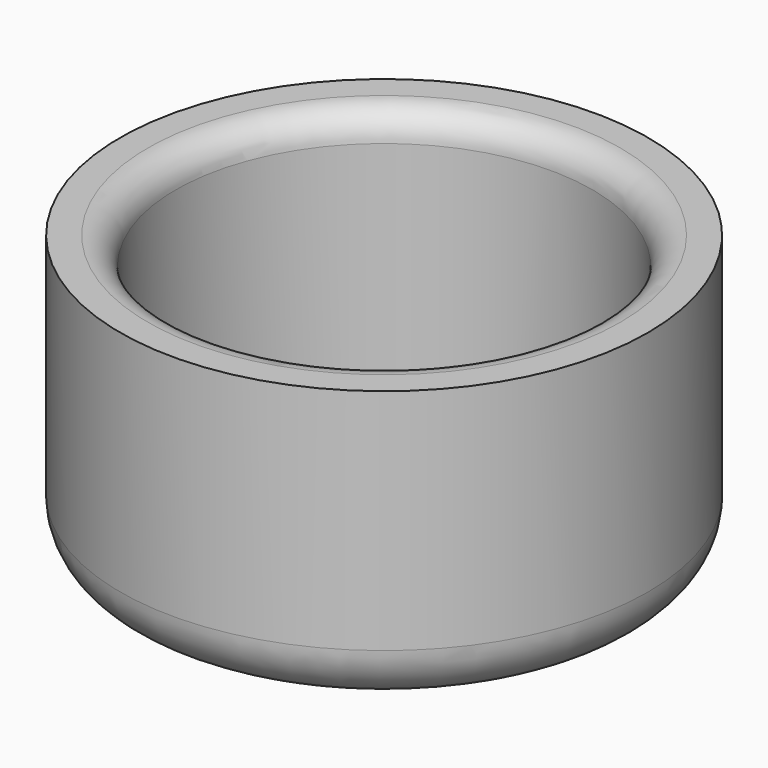
from build123d import *

# Parameters (mm, degrees)
F2_R         = 2
F3_R         = 1
F4_TEXT_SIZE = 3.9131940058
F5_DEPTH     = 1


# Not quite as in the source:
# - Text() gives the source's letters only with a copy of the font that has no kerning and outlines rounded to 1/6400 em; it was checked with that copy


with BuildPart() as f1:
    # F0 (on Front) → F1 (revolve)
    with BuildSketch(Plane.XZ):
        Polygon((7.5, 0), (0, 0), (0, -2), (9.5, -2), (9.5, 8.2183094201), (7.5, 8.2183094201), align=None)
    revolve(axis=Axis((0, 0, -1.6662292182), (0, 0, -1)))

    # F2
    f2_edges = [f1.edges().sort_by_distance(p)[0] for p in [
        (-9.5, 0, -2),
    ]]
    fillet(f2_edges, radius=F2_R)

    # F3
    f3_edges = [f1.edges().sort_by_distance(p)[0] for p in [
        (-7.5, 0, 8.218309),
    ]]
    fillet(f3_edges, radius=F3_R)

    # F4 (on face) → F5 (cut)
    with BuildSketch(Plane(origin=(0, 0, -2), x_dir=(1, 0, 0), z_dir=(0, 0, -1))):
        with Locations((-4.7090166447, 0)):
            Text('Icom', F4_TEXT_SIZE, font='Open Sans', text_align=(TextAlign.LEFT, TextAlign.BOTTOM))
    extrude(amount=-F5_DEPTH, mode=Mode.SUBTRACT)


solid = f1.part
